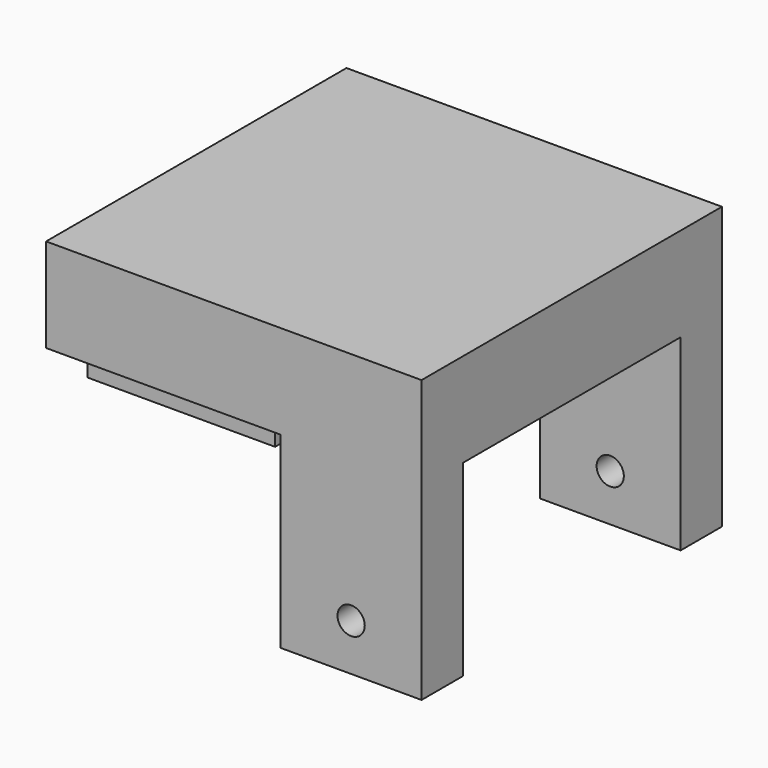
from build123d import *

# Parameters (mm, degrees)
F0_W     = 40
F0_H     = 40
F1_DEPTH = 10
F2_W     = 20
F2_H     = 29
F3_DEPTH = 5
F4_W     = 15
F4_H     = 5.5
F5_DEPTH = 20
F6_R     = 1.45
F7_DEPTH = 53.2


# Not quite as in the source:
# - a feature names something its author has since deleted; it is built from what else it names


with BuildPart() as f1:
    # F0 (on Top) → F1 (new body)
    with BuildSketch(Plane.XY):
        Rectangle(F0_W, F0_H)
    extrude(amount=F1_DEPTH)

    # F2 (on face) → F3 (join)
    with BuildSketch(Plane(origin=(0, 0, 0), x_dir=(1, 0, 0), z_dir=(0, 0, -1))):
        with Locations((-10, 0)):
            Rectangle(F2_W, F2_H)
    extrude(amount=F3_DEPTH)

    # F4 (on face) → F5 (join)
    with BuildSketch(Plane(origin=(0, 0, 0), x_dir=(1, 0, 0), z_dir=(0, 0, -1))):
        with Locations((12.5, 17.25)):
            Rectangle(F4_W, F4_H)
        with Locations((12.5, -17.25)):
            Rectangle(F4_W, F4_H)
    extrude(amount=F5_DEPTH)

    # F6 (on face) → F7 (cut)
    with BuildSketch(Plane.XZ.offset(20)):
        with Locations((12.5, -15)):
            Circle(F6_R)
    extrude(amount=-F7_DEPTH, mode=Mode.SUBTRACT)


solid = f1.part
